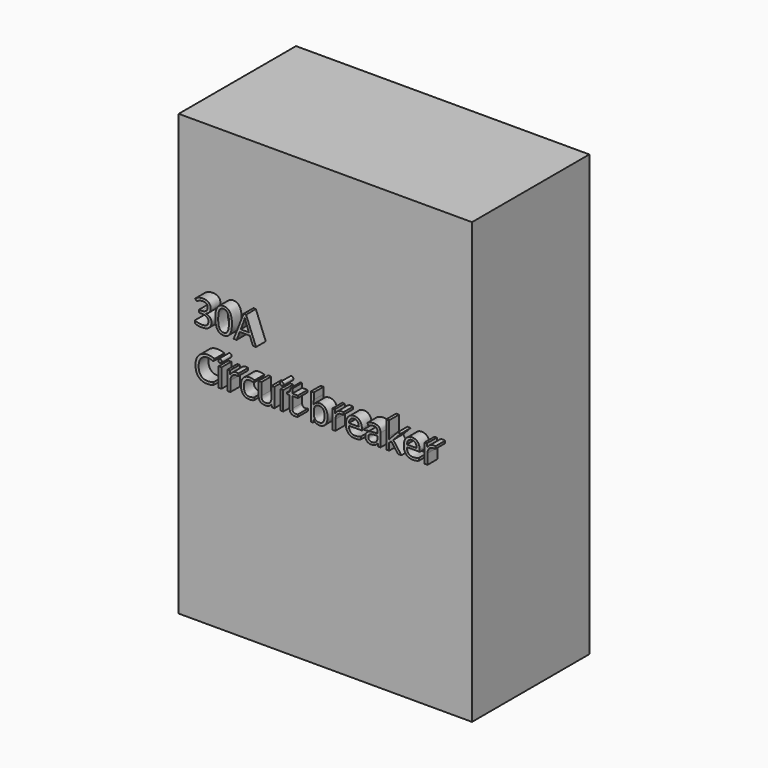
from build123d import *

# Parameters (mm, degrees)
F0_W         = 304.8
F0_H         = 457.2
F1_DEPTH     = 152.4
F2_TEXT_SIZE = 36.6472789576
F3_DEPTH     = 12.7


# Not quite as in the source:
# - Text() gives the source's letters only with a copy of the font that has no kerning and outlines rounded to 1/6400 em; it was checked with that copy


with BuildPart() as f1:
    # F0 (on Front) → F1 (new body)
    with BuildSketch(Plane.XZ):
        Rectangle(F0_W, F0_H)
    extrude(amount=F1_DEPTH)

    # F2 (on face) → F3 (join)
    with BuildSketch(Plane.XZ.offset(152.4)):
        with Locations((-127, 49.8139591505)):
            Text('30A', F2_TEXT_SIZE, font='Open Sans', text_align=(TextAlign.LEFT, TextAlign.BOTTOM))
        with Locations((-127, -0.0263402318)):
            Text('Circuit breaker', F2_TEXT_SIZE, font='Open Sans', text_align=(TextAlign.LEFT, TextAlign.BOTTOM))
    extrude(amount=F3_DEPTH)


solid = f1.part
